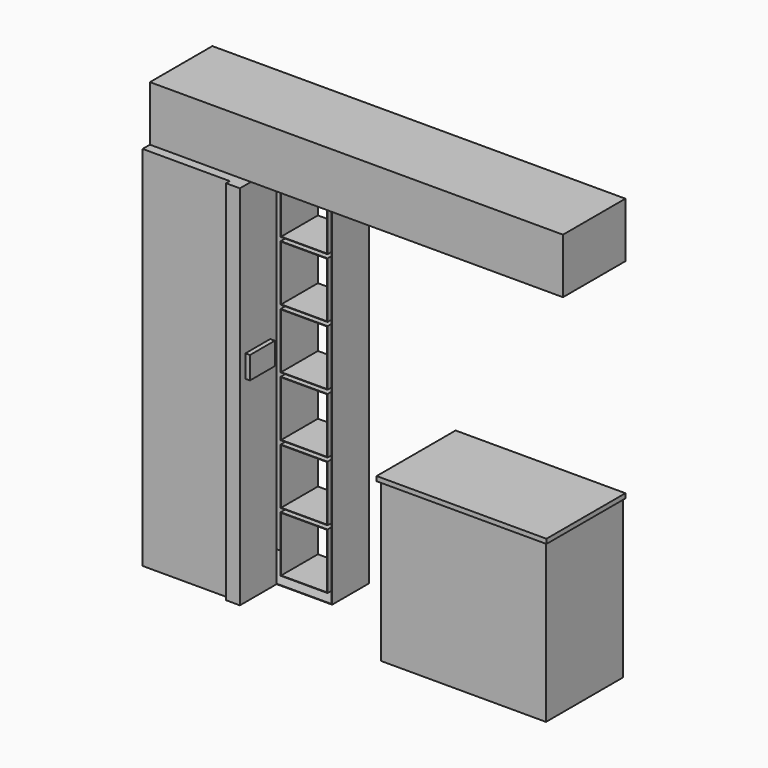
from build123d import *

# Parameters (mm, degrees)
F1_DEPTH = 546.1
F0_W     = 914.4
F0_H     = 876.3
F2_DEPTH = 533.4
F0_W_2   = 482.6
F0_H_2   = 2032
F3_DEPTH = 482.6
F0_W_3   = 76.2
F4_DEPTH = 508
F5_W     = 171.45
F5_H     = 123.825
F6_DEPTH = 25.4
F0_W_4   = 307.34
F0_W_5   = 254
F0_H_3   = 304.8
F0_H_4   = 25.4
F7_DEPTH = 254
F8_DEPTH = 431.8
F9_T     = -2.54


# Not quite as in the source:
# - a shell that OpenCascade refuses in one call is made with other operations: the cavity is built on its own and cut out
# - the program builds the solid bodies; features that only make, move or delete a surface that nothing else refers to are left out


with BuildPart() as f1:
    # F0 (on Front) → F1 (new body)
    with BuildSketch(Plane.XZ):
        Polygon((236.5439048201, -139.7), (249.2439048201, -139.7), (1163.6439048201, -139.7), (1176.3439048201, -139.7), (1176.3439048201, -114.3), (236.5439048201, -114.3), align=None)
    extrude(amount=F1_DEPTH)

    # F0 (on Front) → F2 (join)
    with BuildSketch(Plane.XZ):
        with Locations((706.4439048201, -577.85)):
            Rectangle(F0_W, F0_H)
    extrude(amount=F2_DEPTH)


with BuildPart() as f3:
    # F0 (on Front) → F3 (new body)
    with BuildSketch(Plane.XZ):
        with Locations((-868.3560951799, 0)):
            Rectangle(F0_W_2, F0_H_2)
    extrude(amount=F3_DEPTH)

    # F0 (on Front) → F4 (join)
    with BuildSketch(Plane.XZ):
        with Locations((-588.9560951799, 0)):
            Rectangle(F0_W_3, F0_H_2)
    extrude(amount=F4_DEPTH)

    # F5 (on face) → F6 (join)
    with BuildSketch(Plane.YZ.offset(-550.8560951799)):
        with Locations((-384.175, 134.5584170843)):
            Rectangle(F5_W, F5_H)
    extrude(amount=F6_DEPTH)

    # F0 (on Front) → F7 (join)
    with BuildSketch(Plane.XZ):
        with Locations((-397.1860951799, 0)):
            Rectangle(F0_W_4, F0_H_2)
        Polygon((-525.4560951799, -304.8), (-525.4560951799, 0), (-271.4560951799, 0), (-271.4560951799, -304.8), (-271.4560951799, -330.2), (-271.4560951799, -635), (-271.4560951799, -660.4), (-271.4560951799, -965.2), (-525.4560951799, -965.2), (-525.4560951799, -660.4), (-525.4560951799, -635), (-525.4560951799, -330.2), align=None, mode=Mode.SUBTRACT)
        with Locations((-398.4560951799, 177.8)):
            Rectangle(F0_W_5, F0_H_3, mode=Mode.SUBTRACT)
        with Locations((-398.4560951799, 508)):
            Rectangle(F0_W_5, F0_H_3, mode=Mode.SUBTRACT)
        with Locations((-398.4560951799, 838.2)):
            Rectangle(F0_W_5, F0_H_3, mode=Mode.SUBTRACT)
        with Locations((-398.4560951799, -317.5)):
            Rectangle(F0_W_5, F0_H_4)
        with Locations((-398.4560951799, -647.7)):
            Rectangle(F0_W_5, F0_H_4)
    extrude(amount=F7_DEPTH)

    # F0 (on Front) → F8 (join)
    with BuildSketch(Plane.XZ):
        Polygon((-1109.6560951799, 1320.8), (-1109.6560951799, 1016), (-627.0560951799, 1016), (-550.8560951799, 1016), (-243.5160951799, 1016), (1176.3439048201, 1016), (1176.3439048201, 1320.8), align=None)
    extrude(amount=F8_DEPTH)

    # F9: a shell. OpenCascade refuses it in one call, so the cavity is built on its own and cut out:
    # the body offset inwards by the wall thickness, plus a prism from it out through each open face.
    f9_core = offset(f3.part, amount=F9_T, kind=Kind.INTERSECTION, mode=Mode.PRIVATE)
    f9_exits = [f9_core.faces().sort_by_distance(p)[0] for p in [
        (-399.726095, -251.46, 997.988888),
    ]]
    add(f9_core, mode=Mode.SUBTRACT)
    extrude(f9_exits, amount=-F9_T, mode=Mode.SUBTRACT)


solid = Compound([f1.part, f3.part])
